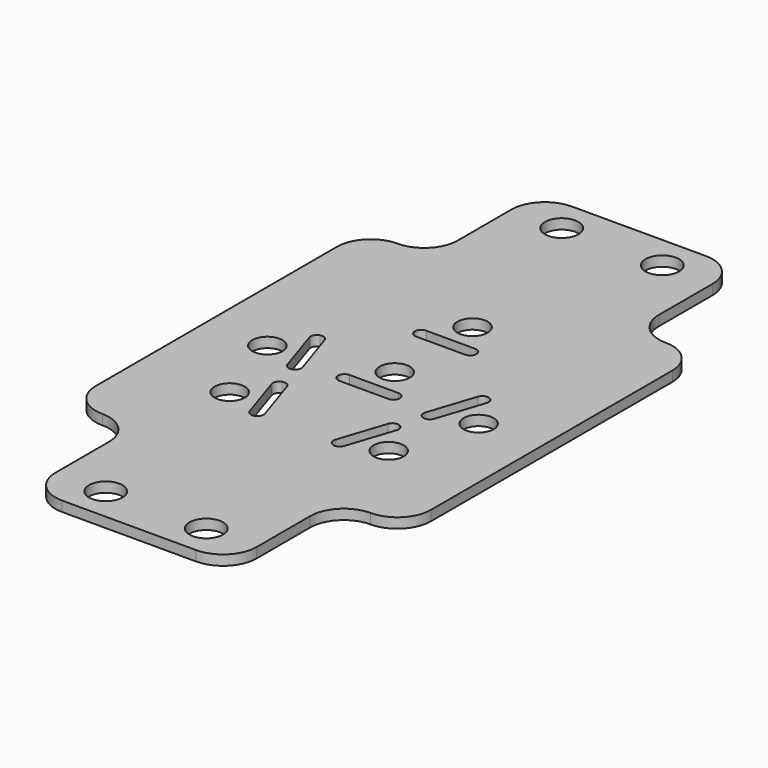
from build123d import *

# Parameters (mm, degrees)
F0_R     = 2.5
F1_DEPTH = 1.5
F2_R     = 4.99999
F3_R     = 2.25
F4_DEPTH = 25
F5_W     = 4.6
F5_H     = 1.9
F5_W_2   = 9.2
F6_DEPTH = 25
F7_R     = 0.94999


# Not quite as in the source:
# - a fillet or chamfer is up to 0.001 mm smaller than in the source, because OpenCascade refuses the exact size


with BuildPart() as f1:
    # F0 (on Top) → F1 (new body)
    with BuildSketch(Plane.XY):
        Polygon((15, 47.5), (-15, 47.5), (-15, 27.5), (-25, 27.5), (-25, -27.5), (-15, -27.5), (-15, -47.5), (15, -47.5), (15, -27.5), (25, -27.5), (25, 27.5), (15, 27.5), align=None)
        with Locations((-7.5, -42.5)):
            Circle(F0_R, mode=Mode.SUBTRACT)
        with Locations((7.5, -42.5)):
            Circle(F0_R, mode=Mode.SUBTRACT)
        with Locations((-7.5, 42.5)):
            Circle(F0_R, mode=Mode.SUBTRACT)
        with Locations((7.5, 42.5)):
            Circle(F0_R, mode=Mode.SUBTRACT)
    extrude(amount=F1_DEPTH)

    # F2 (radius 5 in the source; OpenCascade refuses exactly that, so slightly less here)
    f2_edges = [f1.edges().sort_by_distance(p)[0] for p in [
        (15, 47.5, 0.75),
        (15, 27.5, 0.75),
        (25, 27.5, 0.75),
        (25, -27.5, 0.75),
        (15, -47.5, 0.75),
        (-15, 47.5, 0.75),
        (-15, 27.5, 0.75),
        (-25, 27.5, 0.75),
        (-25, -27.5, 0.75),
        (-15, -47.5, 0.75),
        (-15, -27.5, 0.75),
        (15, -27.5, 0.75),
    ]]
    fillet(f2_edges, radius=F2_R)

    # F3 (on face) → F4 (cut)
    with BuildSketch(Plane.XY.offset(1.5)):
        with Locations((0, 16.5)):
            Circle(F3_R)
        with Locations((0, 2)):
            Circle(F3_R)
        with Locations((15.75, -2.05)):
            Circle(F3_R)
        with Locations((-15.75, -2.05)):
            Circle(F3_R)
        with Locations((11.85, -13.95)):
            Circle(F3_R)
        with Locations((-11.85, -13.95)):
            Circle(F3_R)
    extrude(amount=-F4_DEPTH, mode=Mode.SUBTRACT)

    # F5 (on face) → F6 (cut)
    with BuildSketch(Plane.XY.offset(1.5)):
        with Locations((-2.3, 11.5)):
            Rectangle(F5_W, F5_H)
        with Locations((2.3, 11.5)):
            Rectangle(F5_W, F5_H)
        with Locations((0, -2.8)):
            Rectangle(F5_W_2, F5_H)
        Polygon((-11.7185466768, 4.111970797), (-13.524056425, 3.5202491148), (-10.6588777534, -5.2222191396), (-8.8533680052, -4.6304974575), align=None)
        Polygon((-9.624056425, -8.3797508852), (-6.7588777534, -17.1222191396), (-4.9533680052, -16.5304974575), (-7.8185466768, -7.788029203), align=None)
        Polygon((10.6588777534, -5.2222191396), (13.524056425, 3.5202491148), (11.7185466768, 4.111970797), (8.8533680052, -4.6304974575), align=None)
        Polygon((4.9533680052, -16.5304974575), (6.7588777534, -17.1222191396), (9.624056425, -8.3797508852), (7.8185466768, -7.788029203), align=None)
    extrude(amount=-F6_DEPTH, mode=Mode.SUBTRACT)

    # F7 (radius 0.95 in the source; OpenCascade refuses exactly that, so slightly less here)
    f7_edges = [f1.edges().sort_by_distance(p)[0] for p in [
        (13.524056, 3.520249, 0.75),
        (-8.853368, -4.630497, 0.75),
        (9.624056, -8.379751, 0.75),
        (-4.953368, -16.530497, 0.75),
        (-13.524056, 3.520249, 0.75),
        (-9.624056, -8.379751, 0.75),
        (8.853368, -4.630497, 0.75),
        (4.953368, -16.530497, 0.75),
        (-4.6, 12.45, 0.75),
        (-4.6, -1.85, 0.75),
        (-11.718547, 4.111971, 0.75),
        (11.718547, 4.111971, 0.75),
        (-7.818547, -7.788029, 0.75),
        (7.818547, -7.788029, 0.75),
        (4.6, -1.85, 0.75),
        (4.6, 12.45, 0.75),
        (10.658878, -5.222219, 0.75),
        (-10.658878, -5.222219, 0.75),
        (-4.6, -3.75, 0.75),
        (-4.6, 10.55, 0.75),
        (4.6, 10.55, 0.75),
        (4.6, -3.75, 0.75),
        (-6.758878, -17.122219, 0.75),
        (6.758878, -17.122219, 0.75),
    ]]
    fillet(f7_edges, radius=F7_R)


solid = f1.part
